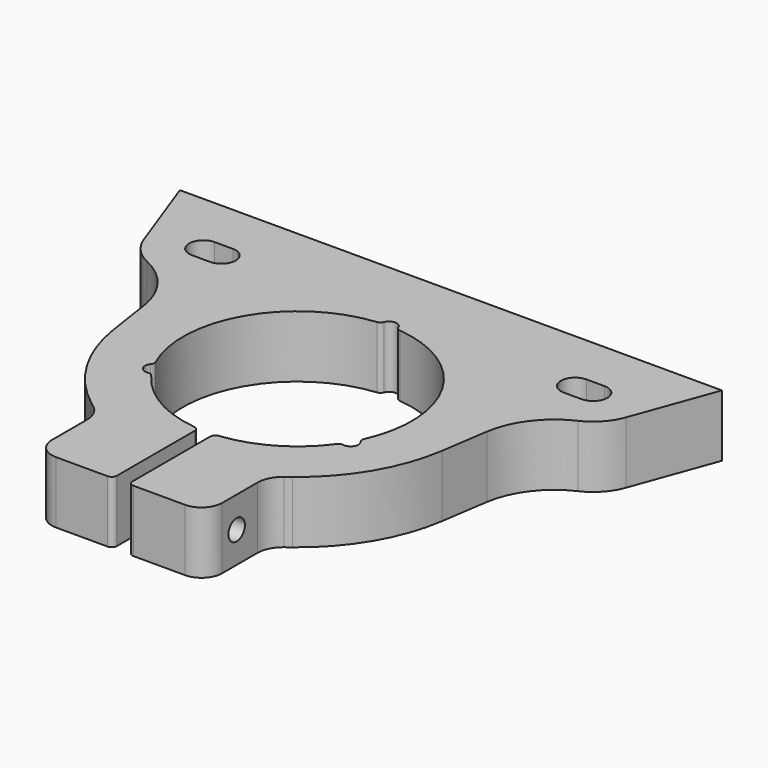
from build123d import *

# Parameters (mm, degrees)
F1_DEPTH = 12
F2_R     = 5
F3_R     = 2
F4_DEPTH = 69.001
F5_R     = 4
F6_R     = 2
F7_DEPTH = 12
F8_R     = 1.5
F9_DEPTH = 25
F10_R    = 1


with BuildPart() as f1:
    # F0 (on Top) → F1 (new body)
    with BuildSketch(Plane.XY):
        with BuildLine():
            Line((52.5, 0), (-52.5, 0))
            Line((-52.5, 0), (-46.6771353676, -15.9990389547))
            ThreePointArc((-46.6771353676, -15.9990389547), (-44.7400164437, -19.1834804046), (-41.7268534535, -21.3775510204))
            ThreePointArc((-41.7268534535, -21.3775510204), (-36.0124674438, -25.9915106654), (-33.1735048367, -32.7652188367))
            Line((-33.1735048367, -32.7652188367), (-31.7911865206, -41.93988096))
            ThreePointArc((-31.7911865206, -41.93988096), (-27.6690936208, -53.5220419681), (-19.5011770908, -62.7102541473))
            Line((-19.5011770908, -62.7102541473), (-16.5, -65))
            Line((-16.5, -65), (-16.5, -80))
            Line((-16.5, -80), (-1.5, -80))
            Line((-1.5, -80), (-1.5, -59.2491515674))
            ThreePointArc((-1.5, -59.2491515674), (0, -15), (1.5, -59.2491515674))
            Line((1.5, -59.2491515674), (1.5, -80))
            Line((1.5, -80), (16.5, -80))
            Line((16.5, -80), (16.5, -65))
            Line((16.5, -65), (19.5011770908, -62.7102541473))
            ThreePointArc((19.5011770908, -62.7102541473), (27.6690936208, -53.5220419681), (31.7911865206, -41.93988096))
            Line((31.7911865206, -41.93988096), (33.1735048367, -32.7652188367))
            ThreePointArc((33.1735048367, -32.7652188367), (36.0124674438, -25.9915106654), (41.7268534535, -21.3775510204))
            ThreePointArc((41.7268534535, -21.3775510204), (44.7400164437, -19.1834804046), (46.6771353676, -15.9990389547))
            Line((46.6771353676, -15.9990389547), (52.5, 0))
        make_face()
        with BuildLine():
            Line((-34.25, -15.5), (-37.75, -15.5))
            ThreePointArc((-37.75, -15.5), (-40.5, -12.75), (-37.75, -10))
            Line((-37.75, -10), (-34.25, -10))
            ThreePointArc((-34.25, -10), (-31.5, -12.75), (-34.25, -15.5))
        make_face(mode=Mode.SUBTRACT)
        with BuildLine():
            ThreePointArc((37.75, -10), (40.5, -12.75), (37.75, -15.5))
            Line((37.75, -15.5), (34.25, -15.5))
            ThreePointArc((34.25, -15.5), (31.5, -12.75), (34.25, -10))
            Line((34.25, -10), (37.75, -10))
        make_face(mode=Mode.SUBTRACT)
    extrude(amount=F1_DEPTH)

    # F2
    f2_edges = [f1.edges().sort_by_distance(p)[0] for p in [
        (-16.5, -65, 6),
        (16.5, -65, 6),
    ]]
    fillet(f2_edges, radius=F2_R)

    # F3 (on face) → F4 (cut, through all)
    with BuildSketch(Plane(origin=(-16.5, 0, 0), x_dir=(0, -1, 0), z_dir=(-1, 0, 0))):
        with Locations((72.5, 6)):
            Circle(F3_R)
    extrude(amount=-F4_DEPTH, mode=Mode.SUBTRACT)

    # F5
    f5_edges = [f1.edges().sort_by_distance(p)[0] for p in [
        (-16.5, -80, 6),
        (16.5, -80, 6),
    ]]
    fillet(f5_edges, radius=F5_R)

    # F6 (on face) → F7 (cut)
    with BuildSketch(Plane(origin=(0, 0, 0), x_dir=(-1, 0, 0), z_dir=(0, 1, 0))):
        with Locations((-36, 6)):
            Circle(F6_R)
        with Locations((36, 6)):
            Circle(F6_R)
    extrude(amount=-F7_DEPTH, mode=Mode.SUBTRACT)

    # F8 (on face) → F9 (cut)
    with BuildSketch(Plane.XY.offset(12)):
        with Locations((0, -15)):
            Circle(F8_R)
        with Locations((-19.1824626938, -48.225)):
            Circle(F8_R)
        with Locations((19.1824626938, -48.225)):
            Circle(F8_R)
    extrude(amount=-F9_DEPTH, mode=Mode.SUBTRACT)

    # F10
    f10_edges = [f1.edges().sort_by_distance(p)[0] for p in [
        (1.49914, -15.05079, 6),
        (-1.49914, -15.05079, 6),
        (-19.888047, -46.901312, 6),
        (-18.388907, -49.497898, 6),
        (18.388907, -49.497898, 6),
        (19.888047, -46.901312, 6),
        (1.5, -59.249152, 6),
        (-1.5, -59.249152, 6),
        (1.5, -80, 6),
        (-1.5, -80, 6),
    ]]
    fillet(f10_edges, radius=F10_R)


solid = f1.part
